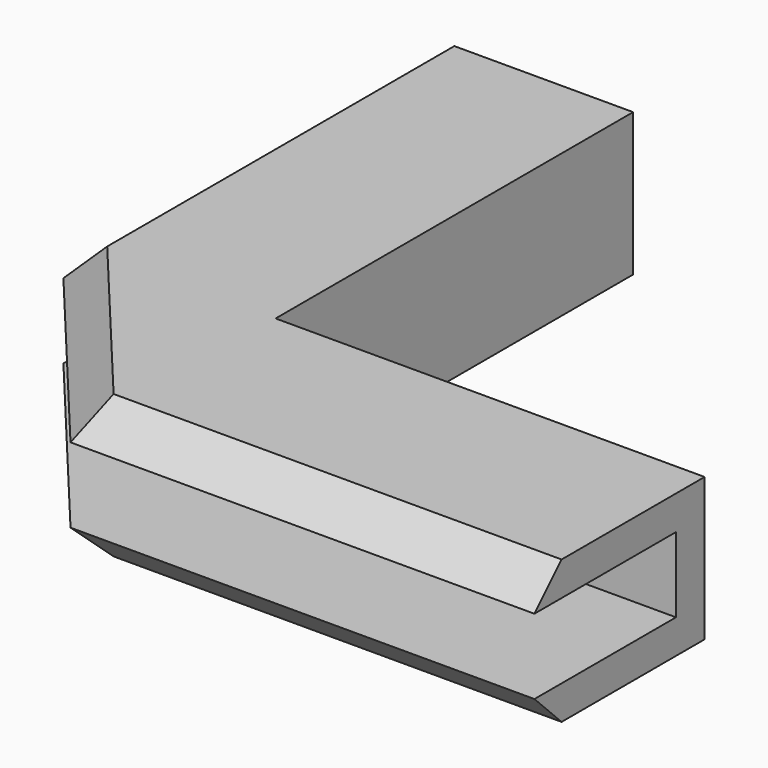
from build123d import *

# Parameters (mm, degrees)
F0_W        = 5
F0_H        = 62.5
F0_H_2      = 5
F0_W_2      = 60
F1_DEPTH    = 10.5
F2_W        = 5
F2_H        = 62.5
F2_W_2      = 25
F2_W_3      = 65
F2_H_2      = 25
F3_DEPTH    = 4.75
F4_W        = 65
F4_H        = 25
F4_W_2      = 5
F4_H_2      = 62.5
F4_W_3      = 25
F5_DEPTH    = 4.75
F6_T1_DEPTH = 88.2168298797
F7_T1_DEPTH = 56.9578285833
F7_T3_DEPTH = 90.7168298797
F7_T5_DEPTH = 88.2168298797
F7_T7_DEPTH = 64.7680782592
F9_D        = 7


# Not quite as in the source:
# - a fillet or chamfer that OpenCascade refuses, or shapes differently, is made with other operations: its cross-section is extruded or revolved along the edge and cut away or added


with BuildPart() as f1:
    # F0 (on Top) → F1 (new body)
    with BuildSketch(Plane.XY):
        with Locations((0, 33.75)):
            Rectangle(F0_W, F0_H)
        Rectangle(F0_W, F0_H_2)
        with Locations((32.5, 0)):
            Rectangle(F0_W_2, F0_H_2)
    extrude(amount=F1_DEPTH)

    # F2 (on face) → F3 (join)
    with BuildSketch(Plane.XY.offset(10.5)):
        with Locations((0, 33.75)):
            Rectangle(F2_W, F2_H)
        Polygon((2.5, 2.5), (-2.5, 2.5), (-2.5, -2.5), (62.5, -2.5), (62.5, 2.5), align=None)
        Polygon((-2.5, -2.5), (-2.5, 2.5), (-27.5, 2.5), (-2.5, -27.5), align=None)
        with Locations((-15, 33.75)):
            Rectangle(F2_W_2, F2_H)
        with Locations((30, -15)):
            Rectangle(F2_W_3, F2_H_2)
    extrude(amount=F3_DEPTH)

    # F4 (on face) → F5 (join)
    with BuildSketch(Plane(origin=(0, 0, 0), x_dir=(1, 0, 0), z_dir=(0, 0, -1))):
        with Locations((30, 15)):
            Rectangle(F4_W, F4_H)
        Polygon((2.5, -2.5), (62.5, -2.5), (62.5, 2.5), (-2.5, 2.5), (-2.5, -2.5), align=None)
        Polygon((-27.5, -2.5), (-2.5, -2.5), (-2.5, 2.5), (-2.5, 27.5), align=None)
        with Locations((0, -33.75)):
            Rectangle(F4_W_2, F4_H_2)
        with Locations((-15, -33.75)):
            Rectangle(F4_W_3, F4_H_2)
    extrude(amount=F5_DEPTH)

    # F6: chamfer of 5 on 1 edges, made by hand

    # F6_s2 → F6_t1 (cut)
    with BuildSketch(Plane.XZ.offset(-77.8584149398)):
        Polygon((-27.5, 10.25), (-22.5, 15.25), (-27.5, 15.25), align=None)
    extrude(amount=F6_T1_DEPTH, mode=Mode.SUBTRACT)

    # F7: chamfer of 5 on 5 edges, made by hand

    # F7_s2 → F7_t1 (cut)
    with BuildSketch(Plane(origin=(-15.7317566489, 18.8781079787, 0), x_dir=(0, 0, 1), z_dir=(0.6401843997, -0.7682212796, 0))):
        Polygon((15.25, 14.5256241898), (10.25, 19.5256241898), (15.25, 19.5256241898), align=None)
    extrude(amount=F7_T1_DEPTH, mode=Mode.SUBTRACT)

    # F7_s4 → F7_t3 (cut)
    with BuildSketch(Plane.YZ.offset(-15.3584149398)):
        Polygon((-22.5, 15.25), (-27.5, 10.25), (-27.5, 15.25), align=None)
        Polygon((-22.5, -4.75), (-27.5, 0.25), (-27.5, -4.75), align=None)
    extrude(amount=F7_T3_DEPTH, mode=Mode.SUBTRACT)

    # F7_s6 → F7_t5 (cut)
    with BuildSketch(Plane.XZ.offset(-77.8584149398)):
        Polygon((-22.5, -4.75), (-27.5, 0.25), (-27.5, -4.75), align=None)
    extrude(amount=F7_T5_DEPTH, mode=Mode.SUBTRACT)

    # F7_s8 → F7_t7 (cut)
    with BuildSketch(Plane(origin=(20.7317566489, -24.8781079787, 0), x_dir=(0, 0, 1), z_dir=(-0.6401843997, 0.7682212796, 0))):
        Polygon((-4.75, -14.5256241898), (0.25, -19.5256241898), (-4.75, -19.5256241898), align=None)
    extrude(amount=F7_T7_DEPTH, mode=Mode.SUBTRACT)

    # F9 (through all)
    with Locations(Plane(origin=(0, 2.5, 0), x_dir=(-1, 0, 0), z_dir=(0, 1, 0))):
        with Locations((-14.02, 5.25)):
            Hole(F9_D / 2)


solid = f1.part
